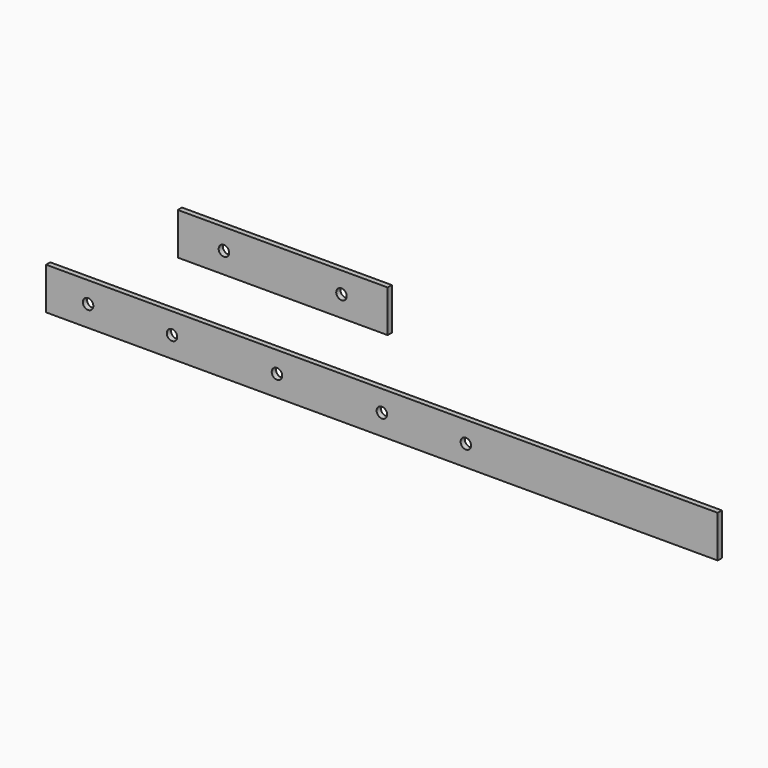
from build123d import *

# Parameters (mm, degrees)
F0_W     = 406.4
F0_H     = 25.4
F0_R     = 3.175
F1_DEPTH = 3.175
F2_W     = 127
F2_H     = 25.4
F2_R     = 3.175
F3_DEPTH = 3.175


# Not quite as in the source:
# - a length typed as a fraction of an inch, garbled in the dataset ("3 / 203.2 mm" for 3/8 in), is restored


with BuildPart() as f1:
    # F0 (on Front) → F1 (new body)
    with BuildSketch(Plane.XZ):
        with Locations((24.4634822011, -11.0960994189)):
            Rectangle(F0_W, F0_H)
        with Locations((-153.3365177989, -11.0960994189)):
            Circle(F0_R, mode=Mode.SUBTRACT)
        with Locations((-102.5365177989, -11.0960994189)):
            Circle(F0_R, mode=Mode.SUBTRACT)
        with Locations((-39.0365177989, -11.0960994189)):
            Circle(F0_R, mode=Mode.SUBTRACT)
        with Locations((24.4634822011, -11.0960994189)):
            Circle(F0_R, mode=Mode.SUBTRACT)
        with Locations((75.2634822011, -11.0960994189)):
            Circle(F0_R, mode=Mode.SUBTRACT)
    extrude(amount=F1_DEPTH)


with BuildPart() as f3:
    # F2 (on Front) → F3 (new body)
    with BuildSketch(Plane.XZ):
        with Locations((-35.56, 43.9982284964)):
            Rectangle(F2_W, F2_H)
        with Locations((-71.12, 43.9982284964)):
            Circle(F2_R, mode=Mode.SUBTRACT)
        with Locations((0, 43.9982284964)):
            Circle(F2_R, mode=Mode.SUBTRACT)
    extrude(amount=F3_DEPTH)


solid = Compound([f1.part, f3.part])
